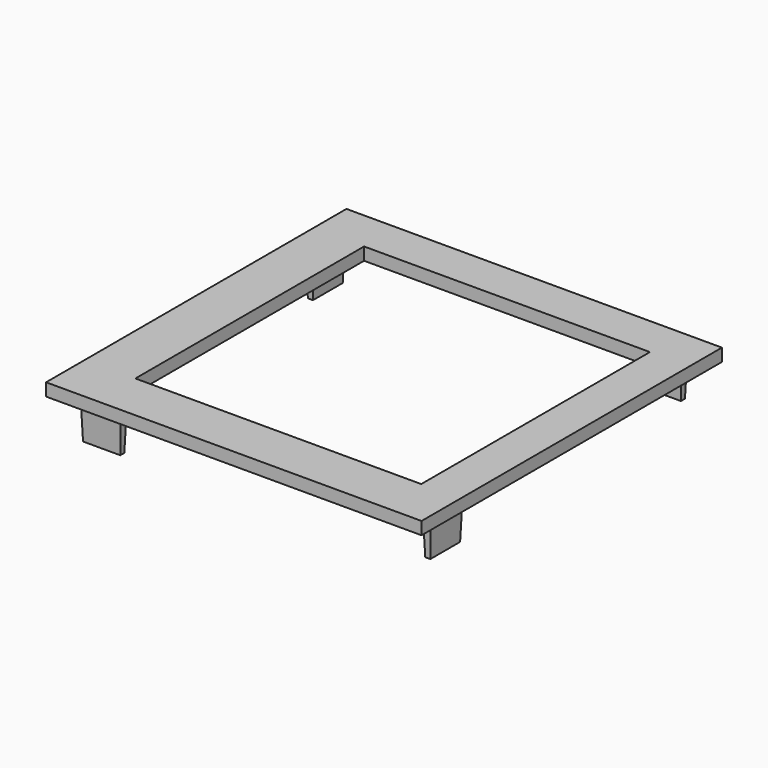
from build123d import *

# Parameters (mm, degrees)
F0_W     = 59.5
F0_H     = 59.5
F0_W_2   = 45.3
F0_H_2   = 45.3
F1_DEPTH = 2
F2_W     = 1.2
F2_H     = 6.3
F2_W_2   = 6.3
F2_H_2   = 1.2
F3_DEPTH = 5.7
F3_TAPER = 2


# Not quite as in the source:
# - a feature names something its author has since deleted; it is built from what else it names


with BuildPart() as f1:
    # F0 (on Top) → F1 (new body)
    with BuildSketch(Plane.XY):
        Rectangle(F0_W, F0_H)
        with Locations((0.8918590039, 0.6)):
            Rectangle(F0_W_2, F0_H_2, mode=Mode.SUBTRACT)
    extrude(amount=F1_DEPTH)

    # F2 (on face) → F3 (join)
    with BuildSketch(Plane(origin=(0, 0, 0), x_dir=(1, 0, 0), z_dir=(0, 0, -1))):
        with Locations((27.3418590039, 22.55)):
            Rectangle(F2_W, F2_H)
        with Locations((22.55, -27.3418590039)):
            Rectangle(F2_W_2, F2_H_2)
        with Locations((-27.3418590039, -22.55)):
            Rectangle(F2_W, F2_H)
        with Locations((-22.55, 27.3418590039)):
            Rectangle(F2_W_2, F2_H_2)
    extrude(amount=F3_DEPTH, taper=F3_TAPER)


solid = f1.part
